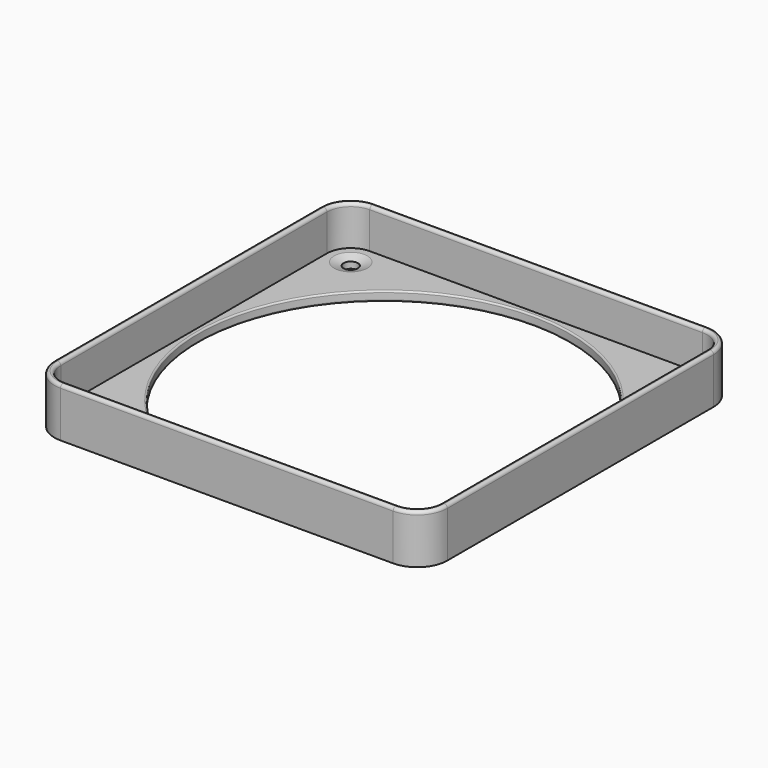
from build123d import *

# Parameters (mm, degrees)
F0_R       = 2.25
F0_R_2     = 58.5
F1_DEPTH   = 3
F2_DEPTH   = 15.5
F3_R       = 0.99999
F4_SIZE2   = 3
F4_SIZE    = 1
F4_2_SIZE2 = 3
F4_2_SIZE  = 1
F4_3_SIZE2 = 3
F4_3_SIZE  = 1
F4_4_SIZE2 = 3
F4_4_SIZE  = 1
F5_R       = 0.5
F6_R       = 0.5


# Not quite as in the source:
# - a fillet or chamfer is up to 0.001 mm smaller than in the source, because OpenCascade refuses the exact size


with BuildPart() as f1:
    # F0 (on Top) → F1 (new body)
    with BuildSketch(Plane.XY):
        with BuildLine():
            Line((52.5, 60), (-52.5, 60))
            ThreePointArc((-52.5, 60), (-57.8033008589, 57.8033008589), (-60, 52.5))
            Line((-60, 52.5), (-60, -52.5))
            ThreePointArc((-60, -52.5), (-57.8033008589, -57.8033008589), (-52.5, -60))
            Line((-52.5, -60), (52.5, -60))
            ThreePointArc((52.5, -60), (57.8033008589, -57.8033008589), (60, -52.5))
            Line((60, -52.5), (60, 52.5))
            ThreePointArc((60, 52.5), (57.8033008589, 57.8033008589), (52.5, 60))
        make_face()
        with Locations((-52.5, -52.5)):
            Circle(F0_R, mode=Mode.SUBTRACT)
        with Locations((52.5, -52.5)):
            Circle(F0_R, mode=Mode.SUBTRACT)
        with Locations((-52.5, 52.5)):
            Circle(F0_R, mode=Mode.SUBTRACT)
        Circle(F0_R_2, mode=Mode.SUBTRACT)
        with Locations((52.5, 52.5)):
            Circle(F0_R, mode=Mode.SUBTRACT)
    extrude(amount=F1_DEPTH)

    # F0 (on Top) → F2 (join)
    with BuildSketch(Plane.XY):
        with BuildLine():
            ThreePointArc((-52.5, 62), (-59.2175144213, 59.2175144213), (-62, 52.5))
            Line((-62, 52.5), (-62, -52.5))
            ThreePointArc((-62, -52.5), (-59.2175144213, -59.2175144213), (-52.5, -62))
            Line((-52.5, -62), (52.5, -62))
            ThreePointArc((52.5, -62), (59.2175144213, -59.2175144213), (62, -52.5))
            Line((62, -52.5), (62, 52.5))
            ThreePointArc((62, 52.5), (59.2175144213, 59.2175144213), (52.5, 62))
            Line((52.5, 62), (-52.5, 62))
        make_face()
        with BuildLine():
            ThreePointArc((-60, 52.5), (-57.8033008589, 57.8033008589), (-52.5, 60))
            Line((-52.5, 60), (52.5, 60))
            ThreePointArc((52.5, 60), (57.8033008589, 57.8033008589), (60, 52.5))
            Line((60, 52.5), (60, -52.5))
            ThreePointArc((60, -52.5), (57.8033008589, -57.8033008589), (52.5, -60))
            Line((52.5, -60), (-52.5, -60))
            ThreePointArc((-52.5, -60), (-57.8033008589, -57.8033008589), (-60, -52.5))
            Line((-60, -52.5), (-60, 52.5))
        make_face(mode=Mode.SUBTRACT)
    extrude(amount=F2_DEPTH)

    # F3 (radius 1 in the source; OpenCascade refuses exactly that, so slightly less here)
    f3_edges = [f1.edges().sort_by_distance(p)[0] for p in [
        (-59.217514, 59.217514, 15.5),
        (-62, 0, 15.5),
        (-59.217514, -59.217514, 15.5),
        (0, -62, 15.5),
        (59.217514, -59.217514, 15.5),
        (62, 0, 15.5),
        (59.217514, 59.217514, 15.5),
        (0, 62, 15.5),
        (-57.803301, 57.803301, 15.5),
        (0, 60, 15.5),
        (57.803301, 57.803301, 15.5),
        (60, 0, 15.5),
        (57.803301, -57.803301, 15.5),
        (0, -60, 15.5),
        (-57.803301, -57.803301, 15.5),
        (-60, 0, 15.5),
    ]]
    fillet(f3_edges, radius=F3_R)

    # F4
    f4_edges = [f1.edges().sort_by_distance(p)[0] for p in [
        (-54.75, 52.5, 3),
    ]]
    f4_side = f1.faces().sort_by_distance((-54.75, 52.5, 1.5))[0]
    chamfer(f4_edges, length=F4_SIZE, length2=F4_SIZE2, reference=f4_side)

    # F4#2
    f4_2_edges = [f1.edges().sort_by_distance(p)[0] for p in [
        (-54.75, -52.5, 3),
    ]]
    f4_2_side = f1.faces().sort_by_distance((-54.75, -52.5, 1.5))[0]
    chamfer(f4_2_edges, length=F4_2_SIZE, length2=F4_2_SIZE2, reference=f4_2_side)

    # F4#3
    f4_3_edges = [f1.edges().sort_by_distance(p)[0] for p in [
        (50.25, 52.5, 3),
    ]]
    f4_3_side = f1.faces().sort_by_distance((50.25, 52.5, 1.5))[0]
    chamfer(f4_3_edges, length=F4_3_SIZE, length2=F4_3_SIZE2, reference=f4_3_side)

    # F4#4
    f4_4_edges = [f1.edges().sort_by_distance(p)[0] for p in [
        (50.25, -52.5, 3),
    ]]
    f4_4_side = f1.faces().sort_by_distance((50.25, -52.5, 1.5))[0]
    chamfer(f4_4_edges, length=F4_4_SIZE, length2=F4_4_SIZE2, reference=f4_4_side)

    # F5
    f5_edges = [f1.edges().sort_by_distance(p)[0] for p in [
        (-58.5, 0, 3),
    ]]
    fillet(f5_edges, radius=F5_R)

    # F6
    f6_edges = [f1.edges().sort_by_distance(p)[0] for p in [
        (-58.5, 0, 0),
    ]]
    fillet(f6_edges, radius=F6_R)


solid = f1.part
